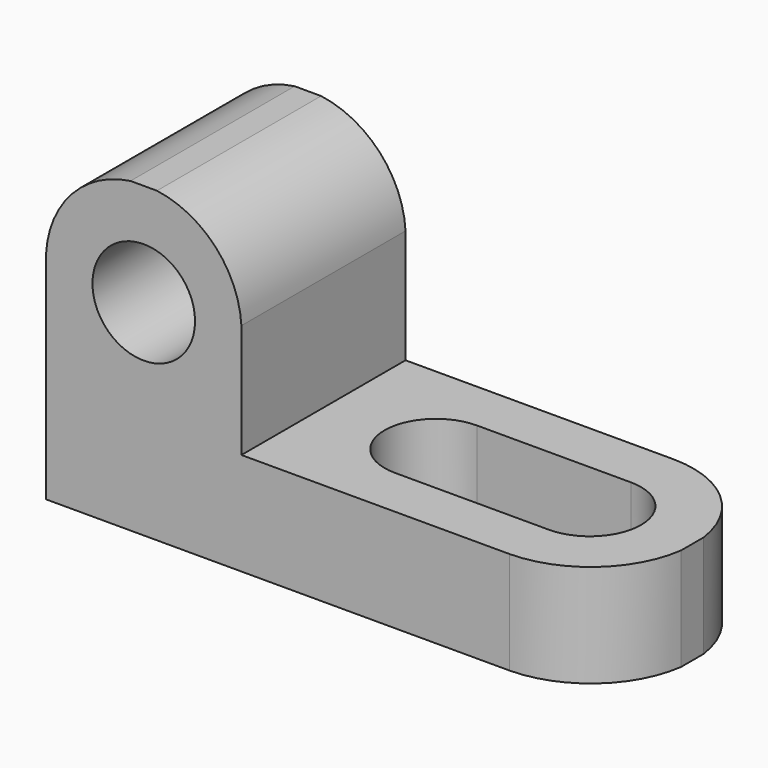
from build123d import *

# Parameters (mm, degrees)
F1_DEPTH = 25.4
F3_DEPTH = 25.401
F5_DEPTH = 12.701


with BuildPart() as f1:
    # F0 (on Front) → F1 (new body)
    with BuildSketch(Plane.XZ):
        Polygon((-6.2236683385, 24.0342710525), (-30.4063118957, 24.0342710525), (-30.4063118957, -14.0657289475), (39.4436881043, -14.0657289475), (39.4436881043, -1.3657289475), (-6.2236683385, -1.3657289475), align=None)
    extrude(amount=F1_DEPTH)

    # F2 (on face) → F3 (cut, through all)
    with BuildSketch(Plane.XZ.offset(25.4)):
        with BuildLine():
            ThreePointArc((-24.6649901171, 11.3342710525), (-18.3149901171, 4.9842710525), (-11.9649901171, 11.3342710525))
            Line((-11.9649901171, 11.3342710525), (-24.6649901171, 11.3342710525))
        make_face()
        with BuildLine():
            Line((-24.6649901171, 11.3342710525), (-11.9649901171, 11.3342710525))
            ThreePointArc((-11.9649901171, 11.3342710525), (-18.3149901171, 17.6842710525), (-24.6649901171, 11.3342710525))
        make_face()
        with BuildLine():
            Line((-6.2236683385, 12.7333663785), (-6.2236683385, 11.3342710525))
            ThreePointArc((-6.2236683385, 11.3342710525), (-6.2034489564, 12.0338187155), (-6.2236683385, 12.7333663785))
        make_face()
        with BuildLine():
            ThreePointArc((-16.678355462, 24.0342710525), (-9.4244440948, 20.258636082), (-6.2236683385, 12.7333663785))
            Line((-6.2236683385, 12.7333663785), (-6.2236683385, 24.0342710525))
            Line((-6.2236683385, 24.0342710525), (-16.678355462, 24.0342710525))
        make_face()
        with BuildLine():
            ThreePointArc((-30.4063118957, 12.7333663785), (-30.4265312777, 12.0338187155), (-30.4063118957, 11.3342710525))
            Line((-30.4063118957, 11.3342710525), (-30.4063118957, 12.7333663785))
        make_face()
        with BuildLine():
            Line((-19.9516247721, 24.0342710525), (-16.678355462, 24.0342710525))
            ThreePointArc((-16.678355462, 24.0342710525), (-18.3149901171, 24.1453598762), (-19.9516247721, 24.0342710525))
        make_face()
        with BuildLine():
            Line((-30.4063118957, 24.0342710525), (-30.4063118957, 12.7333663785))
            ThreePointArc((-30.4063118957, 12.7333663785), (-27.2055361393, 20.258636082), (-19.9516247721, 24.0342710525))
            Line((-19.9516247721, 24.0342710525), (-30.4063118957, 24.0342710525))
        make_face()
    extrude(amount=-F3_DEPTH, mode=Mode.SUBTRACT)

    # F4 (on face) → F5 (cut, through all)
    with BuildSketch(Plane.XY.offset(-1.3657289475)):
        with BuildLine():
            ThreePointArc((33.0936881043, -12.7), (31.2338161649, -8.2098719395), (26.7436881043, -6.35))
            Line((26.7436881043, -6.35), (26.7436881043, -19.05))
            ThreePointArc((26.7436881043, -19.05), (31.2338161649, -17.1901280605), (33.0936881043, -12.7))
        make_face()
        with BuildLine():
            Line((26.7436881043, -19.05), (26.7436881043, -6.35))
            ThreePointArc((26.7436881043, -6.35), (20.3936881043, -12.7), (26.7436881043, -19.05))
        make_face()
        with BuildLine():
            ThreePointArc((26.7436881043, -19.05), (20.3936881043, -12.7), (26.7436881043, -6.35))
            Line((26.7436881043, -6.35), (7.6936881043, -6.35))
            ThreePointArc((7.6936881043, -6.35), (12.1838161649, -8.2098719395), (14.0436881043, -12.7))
            ThreePointArc((14.0436881043, -12.7), (12.1838161649, -17.1901280605), (7.6936881043, -19.05))
            Line((7.6936881043, -19.05), (26.7436881043, -19.05))
        make_face()
        with BuildLine():
            Line((39.4436881043, 0), (26.981144502, 0))
            ThreePointArc((26.981144502, 0), (35.251198478, -3.1641502734), (39.4436881043, -10.9634239866))
            Line((39.4436881043, -10.9634239866), (39.4436881043, 0))
        make_face()
        with BuildLine():
            ThreePointArc((14.0436881043, -12.7), (12.1838161649, -8.2098719395), (7.6936881043, -6.35))
            Line((7.6936881043, -6.35), (7.6936881043, -19.05))
            ThreePointArc((7.6936881043, -19.05), (12.1838161649, -17.1901280605), (14.0436881043, -12.7))
        make_face()
        with BuildLine():
            Line((7.6936881043, -19.05), (7.6936881043, -6.35))
            ThreePointArc((7.6936881043, -6.35), (1.3436881043, -12.7), (7.6936881043, -19.05))
        make_face()
        with BuildLine():
            ThreePointArc((39.4436881043, -14.4365760134), (39.5629712668, -12.7), (39.4436881043, -10.9634239866))
            Line((39.4436881043, -10.9634239866), (39.4436881043, -14.4365760134))
        make_face()
        with BuildLine():
            Line((39.4436881043, -25.4), (39.4436881043, -14.4365760134))
            ThreePointArc((39.4436881043, -14.4365760134), (35.251198478, -22.2358497266), (26.981144502, -25.4))
            Line((26.981144502, -25.4), (39.4436881043, -25.4))
        make_face()
    extrude(amount=-F5_DEPTH, mode=Mode.SUBTRACT)


solid = f1.part
